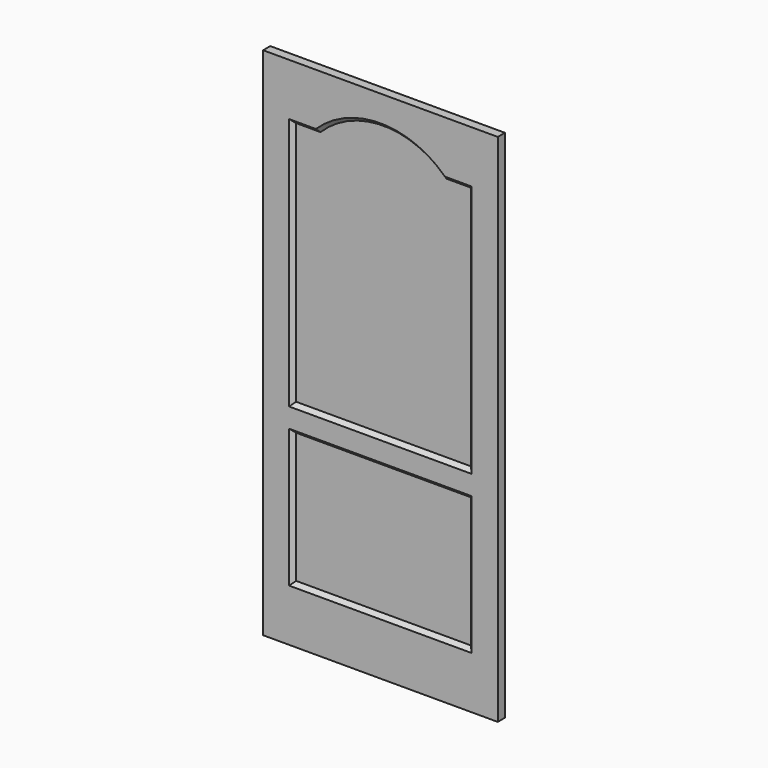
from build123d import *

# Parameters (mm, degrees)
F0_W                     = 914.4
F0_H                     = 2006.6
F0_W_2                   = 711.2
F0_H_2                   = 538.1625
F1_DEPTH                 = 17.4625
F3_DEPTH                 = 15.08125
DRAFT_F3_DRAFTED_ANGLE   = 45
F2_W                     = 711.2
F2_H                     = 538.1625
DRAFT_F3_2_DRAFTED_ANGLE = 45
F5_DEPTH                 = 15.08125
DRAFT_F5_DRAFTED_ANGLE   = 45
F4_W                     = 711.2
F4_H                     = 538.1625
DRAFT_F5_2_DRAFTED_ANGLE = 45


# Not quite as in the source:
# - an extrude with a draft is written as a straight extrude whose walls are then drafted
# - a feature names something its author has since deleted; it is built from what else it names


with BuildPart() as f1:
    # F0 (on Front) → F1 (new body, symmetric)
    with BuildSketch(Plane.XZ):
        with Locations((0, 1003.3)):
            Rectangle(F0_W, F0_H)
        with Locations((0, 472.28125)):
            Rectangle(F0_W_2, F0_H_2, mode=Mode.SUBTRACT)
        with BuildLine():
            Line((355.6, 817.5625), (-355.6, 817.5625))
            Line((-355.6, 817.5625), (-355.6, 1803.4))
            Line((-355.6, 1803.4), (-251.6836974379, 1803.4))
            ThreePointArc((-251.6836974379, 1803.4), (0, 1905), (251.6836974379, 1803.4))
            Line((251.6836974379, 1803.4), (355.6, 1803.4))
            Line((355.6, 1803.4), (355.6, 817.5625))
        make_face(mode=Mode.SUBTRACT)
        with BuildLine():
            Line((-355.6, 1803.4), (-355.6, 817.5625))
            Line((-355.6, 817.5625), (355.6, 817.5625))
            Line((355.6, 817.5625), (355.6, 1803.4))
            Line((355.6, 1803.4), (251.6836974379, 1803.4))
            ThreePointArc((251.6836974379, 1803.4), (0, 1905), (-251.6836974379, 1803.4))
            Line((-251.6836974379, 1803.4), (-355.6, 1803.4))
        make_face()
        with Locations((0, 472.28125)):
            Rectangle(F0_W_2, F0_H_2)
    extrude(amount=F1_DEPTH, both=True)


with BuildPart() as f3_drafted:
    # F2 (on face) → F3 (new body)
    with BuildSketch(Plane(origin=(0, 17.4625, 0), x_dir=(-1, 0, 0), z_dir=(0, 1, 0))):
        with BuildLine():
            Line((-251.6836974379, 1803.4), (-355.6, 1803.4))
            Line((-355.6, 1803.4), (-355.6, 817.5625))
            Line((-355.6, 817.5625), (355.6, 817.5625))
            Line((355.6, 817.5625), (355.6, 1803.4))
            Line((355.6, 1803.4), (251.6836974379, 1803.4))
            ThreePointArc((251.6836974379, 1803.4), (0, 1905), (-251.6836974379, 1803.4))
        make_face()
    extrude(amount=-F3_DEPTH)

    # draft_F3_drafted
    draft_f3_drafted_walls = [f3_drafted.faces().sort_by_distance(p)[0] for p in [
        (303.6418487189, 7.4083333333, 1803.4),
        (355.6, 7.4083333333, 1310.48125),
        (0, 7.4083333333, 817.5625),
        (-355.6, 7.4083333333, 1310.48125),
        (-303.6418487189, 7.4083333333, 1803.4),
        (0, 7.4083333333, 1905),
    ]]
    draft(draft_f3_drafted_walls, neutral_plane=Plane(origin=(0, 17.4625, 0), x_dir=(-1, 0, 0), z_dir=(0, -1, 0)), angle=DRAFT_F3_DRAFTED_ANGLE)


with BuildPart() as f1_1:
    add(f1.part)

    # join_F3_drafted: cut F3_drafted
    add(f3_drafted.part, mode=Mode.SUBTRACT)


with BuildPart() as f3_2_drafted:
    # F2 (on face) → F3, piece 2 (new body)
    with BuildSketch(Plane(origin=(0, 17.4625, 0), x_dir=(-1, 0, 0), z_dir=(0, 1, 0))):
        with Locations((0, 472.28125)):
            Rectangle(F2_W, F2_H)
    extrude(amount=-F3_DEPTH)

    # draft_F3_2_drafted
    draft_f3_2_drafted_walls = [f3_2_drafted.faces().sort_by_distance(p)[0] for p in [
        (-355.6, 7.4083333333, 472.28125),
        (0, 7.4083333333, 741.3625),
        (355.6, 7.4083333333, 472.28125),
        (0, 7.4083333333, 203.2),
    ]]
    draft(draft_f3_2_drafted_walls, neutral_plane=Plane(origin=(0, 17.4625, 0), x_dir=(-1, 0, 0), z_dir=(0, -1, 0)), angle=DRAFT_F3_2_DRAFTED_ANGLE)


with BuildPart() as f1_2:
    add(f1_1.part)

    # join_F3_2_drafted: cut F3_2_drafted
    add(f3_2_drafted.part, mode=Mode.SUBTRACT)


with BuildPart() as f5_drafted:
    # F4 (on face) → F5 (new body)
    with BuildSketch(Plane.XZ.offset(17.4625)):
        with BuildLine():
            Line((-251.6836974379, 1803.4), (-355.6, 1803.4))
            Line((-355.6, 1803.4), (-355.6, 817.5625))
            Line((-355.6, 817.5625), (355.6, 817.5625))
            Line((355.6, 817.5625), (355.6, 1803.4))
            Line((355.6, 1803.4), (251.6836974379, 1803.4))
            ThreePointArc((251.6836974379, 1803.4), (0, 1905), (-251.6836974379, 1803.4))
        make_face()
    extrude(amount=-F5_DEPTH)

    # draft_F5_drafted
    draft_f5_drafted_walls = [f5_drafted.faces().sort_by_distance(p)[0] for p in [
        (0, -7.4083333333, 1905),
        (-303.6418487189, -7.4083333333, 1803.4),
        (-355.6, -7.4083333333, 1310.48125),
        (0, -7.4083333333, 817.5625),
        (355.6, -7.4083333333, 1310.48125),
        (303.6418487189, -7.4083333333, 1803.4),
    ]]
    draft(draft_f5_drafted_walls, neutral_plane=Plane(origin=(0, -17.4625, 0), x_dir=(1, 0, 0), z_dir=(0, 1, 0)), angle=DRAFT_F5_DRAFTED_ANGLE)


with BuildPart() as f1_3:
    add(f1_2.part)

    # join_F5_drafted: cut F5_drafted
    add(f5_drafted.part, mode=Mode.SUBTRACT)


with BuildPart() as f5_2_drafted:
    # F4 (on face) → F5, piece 2 (new body)
    with BuildSketch(Plane.XZ.offset(17.4625)):
        with Locations((0, 472.28125)):
            Rectangle(F4_W, F4_H)
    extrude(amount=-F5_DEPTH)

    # draft_F5_2_drafted
    draft_f5_2_drafted_walls = [f5_2_drafted.faces().sort_by_distance(p)[0] for p in [
        (355.6, -7.4083333333, 472.28125),
        (0, -7.4083333333, 741.3625),
        (-355.6, -7.4083333333, 472.28125),
        (0, -7.4083333333, 203.2),
    ]]
    draft(draft_f5_2_drafted_walls, neutral_plane=Plane(origin=(0, -17.4625, 0), x_dir=(1, 0, 0), z_dir=(0, 1, 0)), angle=DRAFT_F5_2_DRAFTED_ANGLE)


with BuildPart() as f1_4:
    add(f1_3.part)

    # join_F5_2_drafted: cut F5_2_drafted
    add(f5_2_drafted.part, mode=Mode.SUBTRACT)


solid = f1_4.part
